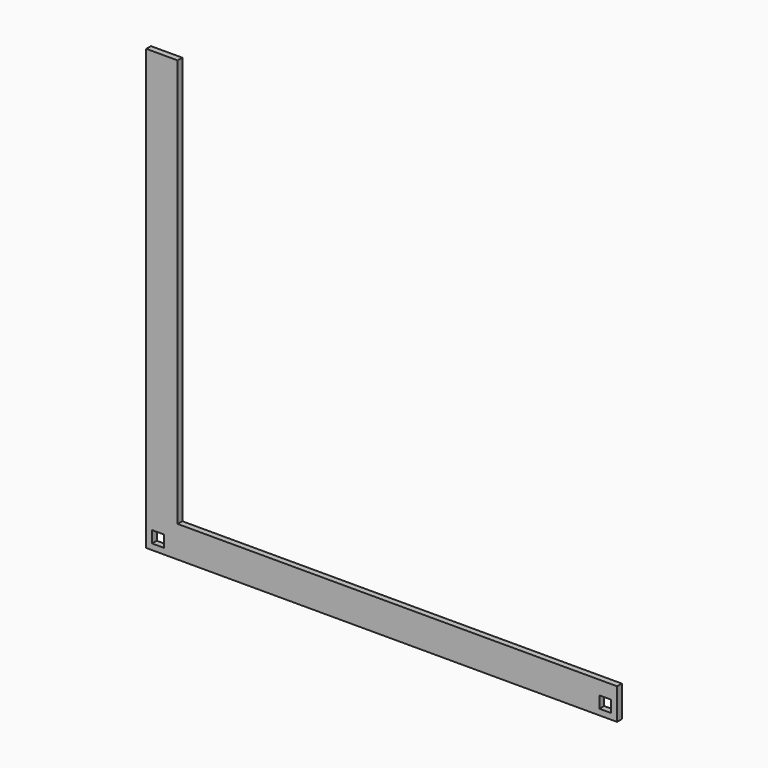
from build123d import *

# Parameters (mm, degrees)
F1_W     = 240
F1_H     = 240
F1_W_2   = 6
F1_H_2   = 6
F1_W_3   = 208
F1_H_3   = 208
F2_DEPTH = 3
F3_DEPTH = 25
F8_W     = 6
F8_H     = 6
F8_W_2   = 16
F8_H_2   = 208
F9_DEPTH = 3.001


with BuildPart() as f2:
    # F1 (on Front) → F2 (new body)
    with BuildSketch(Plane.XZ):
        with Locations((120, 120)):
            Rectangle(F1_W, F1_H)
        with Locations((6, 234)):
            Rectangle(F1_W_2, F1_H_2, mode=Mode.SUBTRACT)
        with Locations((120, 120)):
            Rectangle(F1_W_3, F1_H_3, mode=Mode.SUBTRACT)
        with Locations((6, 234)):
            Rectangle(F1_W_2, F1_H_2)
    extrude(amount=F2_DEPTH)

    # F1 (on Front) → F3 (cut)
    with BuildSketch(Plane.XZ):
        with Locations((6, 234)):
            Rectangle(F1_W_2, F1_H_2)
    extrude(amount=F3_DEPTH, mode=Mode.SUBTRACT)

    # F5: F2 across plane


with BuildPart() as f2_1:
    add(f2.part)
    add(f2.part.mirror(Plane(origin=(120, -1.5, 120), x_dir=(0, -1, 0), z_dir=(-1, 0, 0))), mode=Mode.INTERSECT)

    # F7: F2 across plane


with BuildPart() as f2_2:
    add(f2_1.part)
    add(f2_1.part.mirror(Plane(origin=(120, -1.5, 120), x_dir=(1, 0, 0), z_dir=(0, 0, 1))), mode=Mode.INTERSECT)

    # F8 (on face) → F9 (cut, through all)
    with BuildSketch(Plane.XZ.offset(3)):
        Polygon((240, 240), (0, 240), (0, 224), (16, 224), (224, 224), (240, 224), align=None)
        with Locations((6, 234)):
            Rectangle(F8_W, F8_H, mode=Mode.SUBTRACT)
        with Locations((234, 234)):
            Rectangle(F8_W, F8_H, mode=Mode.SUBTRACT)
        with Locations((232, 120)):
            Rectangle(F8_W_2, F8_H_2)
    extrude(amount=-F9_DEPTH, mode=Mode.SUBTRACT)


solid = f2_2.part
